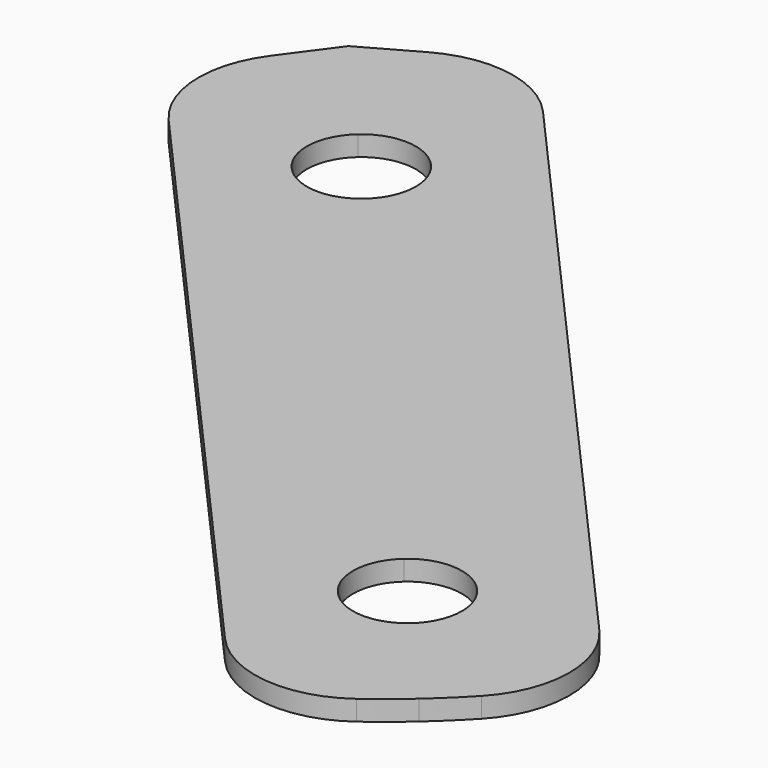
from build123d import *

# Parameters (mm, degrees)
F1_DEPTH = 2.38125


# Not quite as in the source:
# - a feature names something its author has since deleted; it is built from what else it names


with BuildPart() as f1:
    # F0 (on Top) → F1 (new body)
    with BuildSketch(Plane.XY):
        with BuildLine():
            Line((0.0148852749, -0.0168055587), (-12.9522491515, -11.5022529852))
            Line((-12.9522491515, -11.5022529852), (20.5757791682, -49.3555846081))
            ThreePointArc((20.5757791682, -49.3555846081), (28.7380799657, -53.5635383735), (37.6034379496, -51.168656953))
            ThreePointArc((37.6034379496, -51.168656953), (39.8947610083, -49.4030165485), (42.1032952287, -47.5348559574))
            Line((42.1032952287, -47.5348559574), (32.0658696462, -36.2025462971))
            ThreePointArc((32.0658696462, -36.2025462971), (22.9586334857, -35.6506997271), (23.5104800557, -26.5434635666))
            Line((23.5104800557, -26.5434635666), (0.0148852749, -0.0168055587))
        make_face()
        with BuildLine():
            Line((12.9820197013, 11.4686418678), (0.0148852749, -0.0168055587))
            Line((0.0148852749, -0.0168055587), (23.5104800557, -26.5434635666))
            ThreePointArc((23.5104800557, -26.5434635666), (30.4363031351, -25.4899309777), (34.2397748509, -31.3730049319))
            ThreePointArc((34.2397748509, -31.3730049319), (33.6712488051, -34.0211332161), (32.0658696462, -36.2025462971))
            Line((32.0658696462, -36.2025462971), (42.1032952287, -47.5348559574))
            ThreePointArc((42.1032952287, -47.5348559574), (44.2244575032, -45.5680519503), (46.2538460369, -43.5066860011))
            ThreePointArc((46.2538460369, -43.5066860011), (49.7016552964, -34.9953617498), (46.510048021, -26.3846897551))
            Line((46.510048021, -26.3846897551), (12.9820197013, 11.4686418678))
        make_face()
        with BuildLine():
            Line((-48.3172110137, 28.4249868882), (-12.9522491515, -11.5022529852))
            Line((-12.9522491515, -11.5022529852), (0.0148852749, -0.0168055587))
            Line((0.0148852749, -0.0168055587), (0, 0))
            Line((0, 0), (-24.3525459603, 27.4941606857))
            ThreePointArc((-24.3525459603, 27.4941606857), (-33.4597821208, 28.0460072558), (-32.9079355507, 37.1532434163))
            Line((-32.9079355507, 37.1532434163), (-44.6294929424, 50.3869473148))
            Line((-44.6294929424, 50.3869473148), (-49.0520937641, 44.3552682835))
            ThreePointArc((-49.0520937641, 44.3552682835), (-51.4967480049, 36.2604022841), (-48.3172110137, 28.4249868882))
        make_face()
        with BuildLine():
            Line((0, 0), (0.0148852749, -0.0168055587))
            Line((0.0148852749, -0.0168055587), (12.9820197013, 11.4686418678))
            Line((12.9820197013, 11.4686418678), (-22.3829421609, 51.3958817412))
            ThreePointArc((-22.3829421609, 51.3958817412), (-29.7771159339, 55.4982449772), (-38.1079364614, 54.0488936593))
            Line((-38.1079364614, 54.0488936593), (-44.6294929424, 50.3869473148))
            Line((-44.6294929424, 50.3869473148), (-32.9079355507, 37.1532434163))
            ThreePointArc((-32.9079355507, 37.1532434163), (-25.9821124713, 38.2067760052), (-22.1786407555, 32.323702051))
            ThreePointArc((-22.1786407555, 32.323702051), (-22.7471668013, 29.6755737668), (-24.3525459603, 27.4941606857))
            Line((-24.3525459603, 27.4941606857), (0, 0))
        make_face()
    extrude(amount=F1_DEPTH)


solid = f1.part
